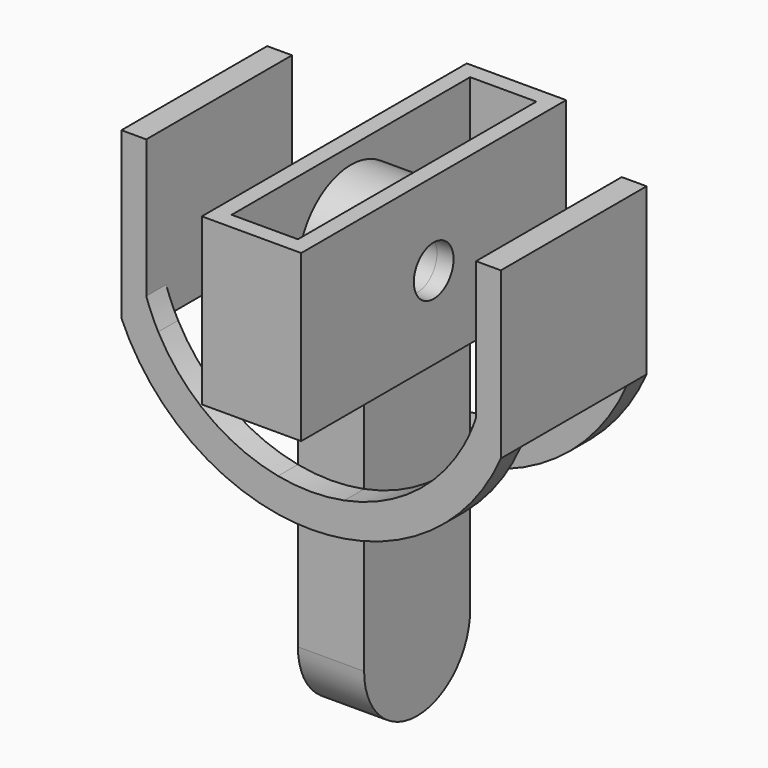
from build123d import *

# Parameters (mm, degrees)
F0_R     = 1.5
F1_DEPTH = 2
F2_W     = 6
F2_H     = 20
F2_W_2   = 4
F2_H_2   = 18
F3_DEPTH = 5
F4_DEPTH = 12.5
F6_DEPTH = 1.5
F7_DEPTH = 8
F8_START = -8
F8_DEPTH = 1.5


# Not quite as in the source:
# - a feature names something its author has since deleted; it is built from what else it names


with BuildPart() as f1:
    # F0 (on Right) → F1 (new body, symmetric)
    with BuildSketch(Plane.YZ):
        with BuildLine():
            ThreePointArc((-4, 0), (0, -4), (4, 0))
            ThreePointArc((4, 0), (0, 4), (-4, 0))
        make_face()
        Circle(F0_R, mode=Mode.SUBTRACT)
        with BuildLine():
            Line((4, -20), (4, 0))
            ThreePointArc((4, 0), (0, -4), (-4, 0))
            Line((-4, 0), (-4, -20))
            ThreePointArc((-4, -20), (0, -16), (4, -20))
        make_face()
        with BuildLine():
            ThreePointArc((-4, -20), (0, -24), (4, -20))
            ThreePointArc((4, -20), (0, -16), (-4, -20))
        make_face()
    extrude(amount=F1_DEPTH, both=True)


with BuildPart() as f3:
    # F2 (on Top) → F3 (new body, symmetric)
    with BuildSketch(Plane.XY):
        Rectangle(F2_W, F2_H)
        Rectangle(F2_W_2, F2_H_2, mode=Mode.SUBTRACT)
    extrude(amount=F3_DEPTH, both=True)

    # F0 (on Right) → F4 (cut, symmetric)
    with BuildSketch(Plane.YZ):
        Circle(F0_R)
    extrude(amount=F4_DEPTH, both=True, mode=Mode.SUBTRACT)


with BuildPart() as f6:
    # F5 (on face) → F6 (new body)
    with BuildSketch(Plane(origin=(0, 4, 0), x_dir=(-1, 0, 0), z_dir=(0, 1, 0))):
        with BuildLine():
            ThreePointArc((-9.9564392374, -3.3345640963), (-10.5, 0), (-9.9564392374, 3.3345640963))
            Line((-9.9564392374, 3.3345640963), (-9.9564392374, 5))
            Line((-9.9564392374, 5), (-11.4564392374, 5))
            Line((-11.4564392374, 5), (-11.4564392374, -5))
            Line((-11.4564392374, -5), (-9.9564392374, -5))
            Line((-9.9564392374, -5), (-9.9564392374, -3.3345640963))
        make_face()
        with BuildLine():
            Line((2, -12.3389626793), (2, -10.307764064))
            ThreePointArc((2, -10.307764064), (0, -10.5), (-2, -10.307764064))
            Line((-2, -10.307764064), (-2, -12.3389626793))
            ThreePointArc((-2, -12.3389626793), (0, -12.5), (2, -12.3389626793))
        make_face()
        with BuildLine():
            ThreePointArc((9.9564392374, 3.3345640963), (10.3632189013, 1.6892880168), (10.5, 0))
            ThreePointArc((10.5, 0), (10.3632189013, -1.6892880168), (9.9564392374, -3.3345640963))
            Line((9.9564392374, -3.3345640963), (9.9564392374, -5))
            Line((9.9564392374, -5), (11.4564392374, -5))
            Line((11.4564392374, -5), (11.4564392374, 5))
            Line((11.4564392374, 5), (9.9564392374, 5))
            Line((9.9564392374, 5), (9.9564392374, 3.3345640963))
        make_face()
        with BuildLine():
            ThreePointArc((9.9564392374, -3.3345640963), (10.3632189013, -1.6892880168), (10.5, 0))
            ThreePointArc((10.5, 0), (10.3632189013, 1.6892880168), (9.9564392374, 3.3345640963))
            Line((9.9564392374, 3.3345640963), (9.9564392374, -3.3345640963))
        make_face()
        with BuildLine():
            Line((9.9564392374, -5), (9.2330926563, -5))
            ThreePointArc((9.2330926563, -5), (6.2119789517, -8.4653007923), (2, -10.307764064))
            Line((2, -10.307764064), (2, -12.3389626793))
            ThreePointArc((2, -12.3389626793), (7.6638131853, -9.8750173398), (11.4564392374, -5))
            Line((11.4564392374, -5), (9.9564392374, -5))
        make_face()
        with BuildLine():
            Line((-2, -12.3389626793), (-2, -10.307764064))
            ThreePointArc((-2, -10.307764064), (-6.2119789517, -8.4653007923), (-9.2330926563, -5))
            Line((-9.2330926563, -5), (-9.9564392374, -5))
            Line((-9.9564392374, -5), (-11.4564392374, -5))
            ThreePointArc((-11.4564392374, -5), (-7.6638131853, -9.8750173398), (-2, -12.3389626793))
        make_face()
        with BuildLine():
            ThreePointArc((-9.2330926563, -5), (-9.6308334407, -4.1829471952), (-9.9564392374, -3.3345640963))
            Line((-9.9564392374, -3.3345640963), (-9.9564392374, -5))
            Line((-9.9564392374, -5), (-9.2330926563, -5))
        make_face()
        with BuildLine():
            Line((-9.9564392374, -3.3345640963), (-9.9564392374, 3.3345640963))
            ThreePointArc((-9.9564392374, 3.3345640963), (-10.5, 0), (-9.9564392374, -3.3345640963))
        make_face()
        with BuildLine():
            Line((9.9564392374, -5), (9.9564392374, -3.3345640963))
            ThreePointArc((9.9564392374, -3.3345640963), (9.6308334407, -4.1829471952), (9.2330926563, -5))
            Line((9.2330926563, -5), (9.9564392374, -5))
        make_face()
    extrude(amount=F6_DEPTH)

    # F5 (on face) → F7 (join, through all)
    with BuildSketch(Plane(origin=(0, 4, 0), x_dir=(-1, 0, 0), z_dir=(0, 1, 0))):
        with BuildLine():
            ThreePointArc((9.9564392374, 3.3345640963), (10.3632189013, 1.6892880168), (10.5, 0))
            ThreePointArc((10.5, 0), (10.3632189013, -1.6892880168), (9.9564392374, -3.3345640963))
            Line((9.9564392374, -3.3345640963), (9.9564392374, -5))
            Line((9.9564392374, -5), (11.4564392374, -5))
            Line((11.4564392374, -5), (11.4564392374, 5))
            Line((11.4564392374, 5), (9.9564392374, 5))
            Line((9.9564392374, 5), (9.9564392374, 3.3345640963))
        make_face()
        with BuildLine():
            ThreePointArc((-9.9564392374, -3.3345640963), (-10.5, 0), (-9.9564392374, 3.3345640963))
            Line((-9.9564392374, 3.3345640963), (-9.9564392374, 5))
            Line((-9.9564392374, 5), (-11.4564392374, 5))
            Line((-11.4564392374, 5), (-11.4564392374, -5))
            Line((-11.4564392374, -5), (-9.9564392374, -5))
            Line((-9.9564392374, -5), (-9.9564392374, -3.3345640963))
        make_face()
        with BuildLine():
            ThreePointArc((9.9564392374, -3.3345640963), (10.3632189013, -1.6892880168), (10.5, 0))
            ThreePointArc((10.5, 0), (10.3632189013, 1.6892880168), (9.9564392374, 3.3345640963))
            Line((9.9564392374, 3.3345640963), (9.9564392374, -3.3345640963))
        make_face()
        with BuildLine():
            Line((-9.9564392374, -3.3345640963), (-9.9564392374, 3.3345640963))
            ThreePointArc((-9.9564392374, 3.3345640963), (-10.5, 0), (-9.9564392374, -3.3345640963))
        make_face()
    extrude(amount=-F7_DEPTH)

    # F5 (on face) → F8 (join)
    with BuildSketch(Plane(origin=(0, 4, 0), x_dir=(-1, 0, 0), z_dir=(0, 1, 0)).offset(F8_START)):
        with BuildLine():
            ThreePointArc((-9.9564392374, -3.3345640963), (-10.5, 0), (-9.9564392374, 3.3345640963))
            Line((-9.9564392374, 3.3345640963), (-9.9564392374, 5))
            Line((-9.9564392374, 5), (-11.4564392374, 5))
            Line((-11.4564392374, 5), (-11.4564392374, -5))
            Line((-11.4564392374, -5), (-9.9564392374, -5))
            Line((-9.9564392374, -5), (-9.9564392374, -3.3345640963))
        make_face()
        with BuildLine():
            ThreePointArc((9.9564392374, 3.3345640963), (10.3632189013, 1.6892880168), (10.5, 0))
            ThreePointArc((10.5, 0), (10.3632189013, -1.6892880168), (9.9564392374, -3.3345640963))
            Line((9.9564392374, -3.3345640963), (9.9564392374, -5))
            Line((9.9564392374, -5), (11.4564392374, -5))
            Line((11.4564392374, -5), (11.4564392374, 5))
            Line((11.4564392374, 5), (9.9564392374, 5))
            Line((9.9564392374, 5), (9.9564392374, 3.3345640963))
        make_face()
        with BuildLine():
            Line((9.9564392374, -5), (9.2330926563, -5))
            ThreePointArc((9.2330926563, -5), (6.2119789517, -8.4653007923), (2, -10.307764064))
            Line((2, -10.307764064), (2, -12.3389626793))
            ThreePointArc((2, -12.3389626793), (7.6638131853, -9.8750173398), (11.4564392374, -5))
            Line((11.4564392374, -5), (9.9564392374, -5))
        make_face()
        with BuildLine():
            Line((-2, -12.3389626793), (-2, -10.307764064))
            ThreePointArc((-2, -10.307764064), (-6.2119789517, -8.4653007923), (-9.2330926563, -5))
            Line((-9.2330926563, -5), (-9.9564392374, -5))
            Line((-9.9564392374, -5), (-11.4564392374, -5))
            ThreePointArc((-11.4564392374, -5), (-7.6638131853, -9.8750173398), (-2, -12.3389626793))
        make_face()
        with BuildLine():
            Line((2, -12.3389626793), (2, -10.307764064))
            ThreePointArc((2, -10.307764064), (0, -10.5), (-2, -10.307764064))
            Line((-2, -10.307764064), (-2, -12.3389626793))
            ThreePointArc((-2, -12.3389626793), (0, -12.5), (2, -12.3389626793))
        make_face()
        with BuildLine():
            ThreePointArc((9.9564392374, -3.3345640963), (10.3632189013, -1.6892880168), (10.5, 0))
            ThreePointArc((10.5, 0), (10.3632189013, 1.6892880168), (9.9564392374, 3.3345640963))
            Line((9.9564392374, 3.3345640963), (9.9564392374, -3.3345640963))
        make_face()
        with BuildLine():
            Line((-9.9564392374, -3.3345640963), (-9.9564392374, 3.3345640963))
            ThreePointArc((-9.9564392374, 3.3345640963), (-10.5, 0), (-9.9564392374, -3.3345640963))
        make_face()
        with BuildLine():
            Line((9.9564392374, -5), (9.9564392374, -3.3345640963))
            ThreePointArc((9.9564392374, -3.3345640963), (9.6308334407, -4.1829471952), (9.2330926563, -5))
            Line((9.2330926563, -5), (9.9564392374, -5))
        make_face()
        with BuildLine():
            ThreePointArc((-9.2330926563, -5), (-9.6308334407, -4.1829471952), (-9.9564392374, -3.3345640963))
            Line((-9.9564392374, -3.3345640963), (-9.9564392374, -5))
            Line((-9.9564392374, -5), (-9.2330926563, -5))
        make_face()
    extrude(amount=-F8_DEPTH)


solid = Compound([f1.part, f3.part, f6.part])
